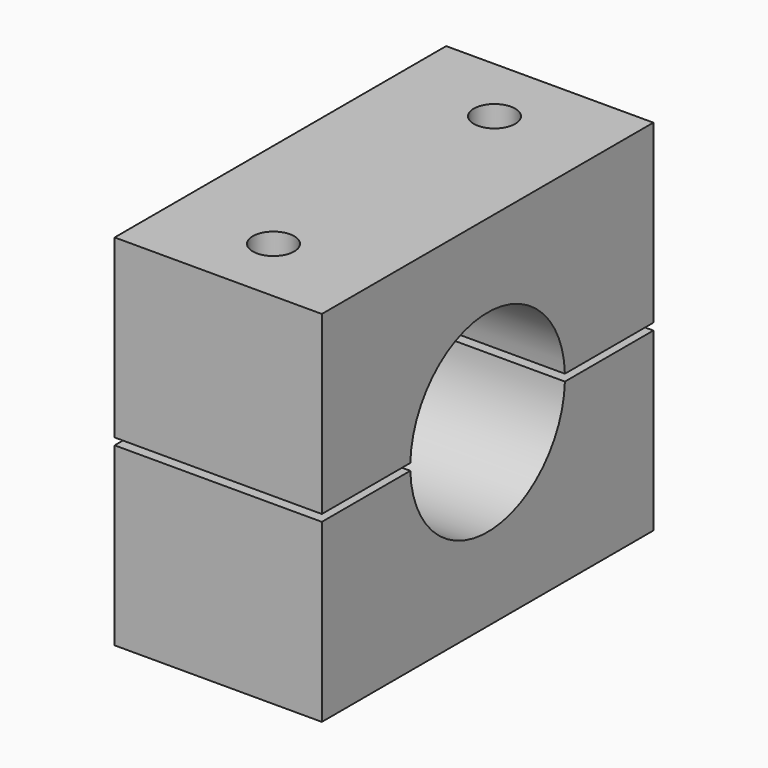
from build123d import *

# Parameters (mm, degrees)
F1_DEPTH = 30
F2_R     = 3
F3_DEPTH = 52


with BuildPart() as f1:
    # F0 (on Right) → F1 (new body)
    with BuildSketch(Plane.YZ):
        with BuildLine():
            Line((-30, -26), (30, -26))
            Line((30, -26), (30, -0.5))
            Line((30, -0.5), (13.9910685796, -0.5))
            ThreePointArc((13.9910685796, -0.5), (0, -14), (-13.9910685796, -0.5))
            Line((-13.9910685796, -0.5), (-30, -0.5))
            Line((-30, -0.5), (-30, -26))
        make_face()
    extrude(amount=F1_DEPTH)


with BuildPart() as f1b:
    # F0 (on Right) → F1, piece 2 (new body)
    with BuildSketch(Plane.YZ):
        with BuildLine():
            Line((30, 0.5), (30, 26))
            Line((30, 26), (-30, 26))
            Line((-30, 26), (-30, 0.5))
            Line((-30, 0.5), (-13.9910685796, 0.5))
            ThreePointArc((-13.9910685796, 0.5), (0, 14), (13.9910685796, 0.5))
            Line((13.9910685796, 0.5), (30, 0.5))
        make_face()
    extrude(amount=F1_DEPTH)

    # F2 (on face) → F3 (cut)
    with BuildSketch(Plane.XY.offset(26)):
        with Locations((15, 20)):
            Circle(F2_R)
        with Locations((15, -20)):
            Circle(F2_R)
    extrude(amount=-F3_DEPTH, mode=Mode.SUBTRACT)


solid = Compound([f1.part, f1b.part])
